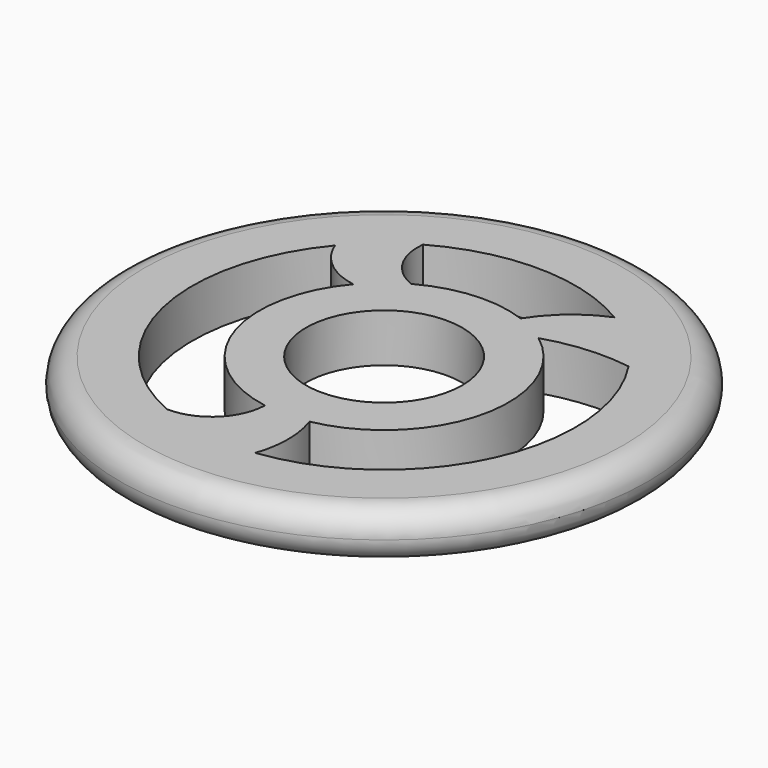
from build123d import *

# Parameters (mm, degrees)
F0_R     = 38.1945033512
F0_R_2   = 11.3
F1_DEPTH = 7
F2_R     = 3.49999


# Not quite as in the source:
# - a fillet or chamfer is up to 0.001 mm smaller than in the source, because OpenCascade refuses the exact size


with BuildPart() as f1:
    # F0 (on Top) → F1 (new body)
    with BuildSketch(Plane.XY):
        Circle(F0_R)
        with BuildLine():
            ThreePointArc((-11.1190587191, -25.3990096631), (-26.9847609568, -6.3691313979), (-21.3025923236, 17.7466255653))
            ThreePointArc((-21.3025923236, 17.7466255653), (-18.3465502514, 13.6852419499), (-13.7577746625, 11.6416763896))
            ThreePointArc((-13.7577746625, 11.6416763896), (-16.9304092047, -6.1778828887), (-3.0268251987, -17.7663536507))
            ThreePointArc((-3.0268251987, -17.7663536507), (-5.4906522747, -23.2602441725), (-11.1190587191, -25.3990096631))
        make_face(mode=Mode.SUBTRACT)
        with BuildLine():
            ThreePointArc((3.3689917925, -27.5207749339), (4.1908869079, -22.6127160748), (3.3689917925, -17.7046572157))
            ThreePointArc((3.3689917925, -17.7046572157), (17.5564618696, -4.0713191283), (10.8174583905, 14.4148391179))
            ThreePointArc((10.8174583905, 14.4148391179), (16.8916900663, 15.5906448864), (23.0748101796, 15.3719320138))
            ThreePointArc((23.0748101796, 15.3719320138), (25.1945379599, -11.5749045633), (3.3689917925, -27.5207749339))
        make_face(mode=Mode.SUBTRACT)
        Circle(F0_R_2, mode=Mode.SUBTRACT)
        with BuildLine():
            ThreePointArc((-8.6949064417, 15.7861836678), (-12.603803519, 19.1055384299), (-13.6713432148, 24.1213086993))
            ThreePointArc((-13.6713432148, 24.1213086993), (0.373914134, 27.7236964866), (14.3169083029, 23.7438264673))
            ThreePointArc((14.3169083029, 23.7438264673), (9.7472249081, 20.9497927504), (6.2279462514, 16.9120571875))
            ThreePointArc((6.2279462514, 16.9120571875), (-1.3558653844, 17.9712721276), (-8.6949064417, 15.7861836678))
        make_face(mode=Mode.SUBTRACT)
    extrude(amount=F1_DEPTH)

    # F2 (radius 3.5 in the source; OpenCascade refuses exactly that, so slightly less here)
    f2_edges = [f1.edges().sort_by_distance(p)[0] for p in [
        (-38.194503, 0, 7),
        (-38.194503, 0, 0),
    ]]
    fillet(f2_edges, radius=F2_R)


solid = f1.part
